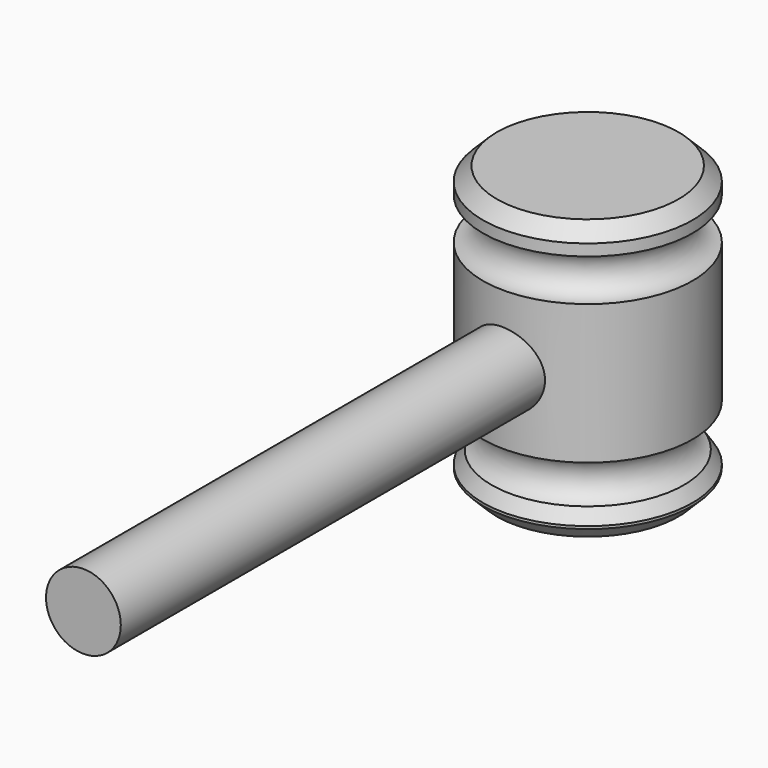
from build123d import *

# Parameters (mm, degrees)
F2_R     = 13.5980918735
F3_DEPTH = 228.6


# Not quite as in the source:
# - a fillet or chamfer that OpenCascade refuses, or shapes differently, is made with other operations: its cross-section is extruded or revolved along the edge and cut away or added


with BuildPart() as f1:
    # F0 (on Front) → F1 (revolve)
    with BuildSketch(Plane.XZ):
        with BuildLine():
            Line((25.3469641268, 61.8318257093), (-12.7530358732, 61.8318257093))
            Line((-12.7530358732, 61.8318257093), (-12.7530358732, 52.5684214187))
            ThreePointArc((-12.7530358732, 52.5684214187), (-5.1330358732, 44.9484214187), (-12.7530358732, 37.3284214187))
            Line((-12.7530358732, 37.3284214187), (-12.7530358732, -13.4300431368))
            ThreePointArc((-12.7530358732, -13.4300431368), (-4.6335244682, -21.5495545417), (-12.7530358732, -29.6690659466))
            Line((-12.7530358732, -29.6690659466), (-12.7530358732, -39.7681742907))
            Line((-12.7530358732, -39.7681742907), (25.3469641268, -39.7681742907))
            Line((25.3469641268, -39.7681742907), (25.3469641268, 61.8318257093))
        make_face()
    revolve(axis=Axis((25.3469641268, 0, 11.0318257093), (0, 0, -1)))

    # F2 (on Front) → F3 (join)
    with BuildSketch(Plane.XZ):
        with Locations((24.8341448605, 11.9163831696)):
            Circle(F2_R)
    extrude(amount=F3_DEPTH)

    # F4: chamfer of 5.08 on 4 edges, made by hand

    # F4_s1 → F4_t2 (revolve, cut)
    with BuildSketch(Plane.XZ):
        Polygon((-7.6730358732, 61.8318257093), (-12.7530358732, 56.7518257093), (-12.7530358732, 61.8318257093), align=None)
    revolve(axis=Axis((25.3469641268, 0, 61.8318257093), (0, 0, -1)), mode=Mode.SUBTRACT)

    # F4_s3 → F4_t4 (revolve, cut)
    with BuildSketch(Plane.XZ):
        with BuildLine():
            Line((-9.6281385439, -29.0436510274), (-12.7530358732, -33.7323580503))
            Line((-12.7530358732, -33.7323580503), (-12.7530358732, -29.6690659466))
            ThreePointArc((-12.7530358732, -29.6690659466), (-11.0871747515, -29.4963383048), (-9.6281385439, -29.0436510274))
        make_face()
    revolve(axis=Axis((25.3469641268, 0, -29.6690659466), (0, 0, -1)), mode=Mode.SUBTRACT)

    # F4_s5 → F4_t6 (revolve, cut)
    with BuildSketch(Plane.XZ):
        Polygon((-12.7530358732, -34.6881742907), (-7.6730358732, -39.7681742907), (-12.7530358732, -39.7681742907), align=None)
    revolve(axis=Axis((25.3469641268, 0, -39.7681742907), (0, 0, -1)), mode=Mode.SUBTRACT)


solid = f1.part
